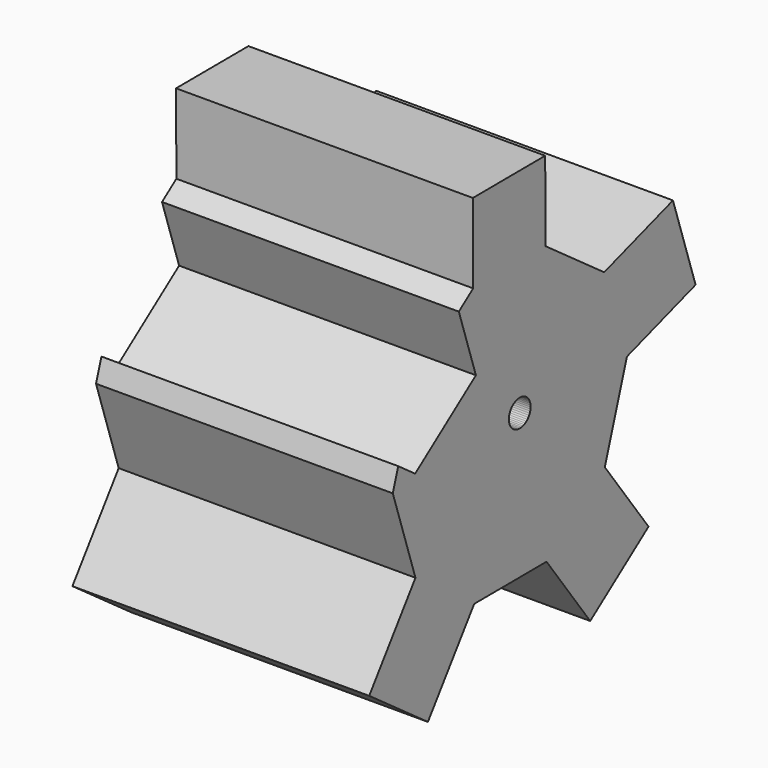
from build123d import *

# Parameters (mm, degrees)
F1_DEPTH = 59.967
F2_DEPTH = 16.11587
F3_DEPTH = 18.27724
F4_DEPTH = 18.65924
F5_DEPTH = 20.01095


with BuildPart() as f1:
    # F0 (on Right) → F1 (new body)
    with BuildSketch(Plane.YZ):
        Polygon((19.3016365517, 25.5114351168), (34.1311297964, 14.8414346621), (52.4001107586, 14.9257803925), (67.1304496505, 25.7322551057), (72.6956576812, 43.1331527599), (66.9700145375, 60.481921886), (52.1405212928, 71.1519223406), (33.8715403306, 71.0675766103), (30.248601096, 68.4097150693), (34.5660174948, 55.3278902953), (19.2159686951, 44.0667838525), (14.944761002, 47.1399696503), (13.575993408, 42.8602042428), align=None)
        Polygon((43.3843278169, 42.5439793365), (43.2058611327, 42.8390985452), (43.0657899565, 43.1542584575), (42.9663232941, 43.4844888132), (42.9090297944, 43.8245816823), (42.8948130101, 44.1691735971), (42.9238971483, 44.5128301373), (42.9958235348, 44.850131634), (43.1094578475, 45.175758641), (43.2630080055, 45.484575826), (43.454052431, 45.7717129574), (43.6795782392, 46.0326417111), (43.9360287536, 46.2632470849), (44.2193595962, 46.4598922942), (44.5251024704, 46.6194761267), (44.8484356285, 46.7394818499), (45.1842599134, 46.8180169019), (45.5272791756, 46.853842738), (45.8720837963, 46.8463943634), (46.2132360006, 46.7957892434), (46.5453556147, 46.7028254509), (46.8632049136, 46.5689690806), (47.1617712242, 46.3963311273), (47.4363459773, 46.1876341948), (47.6825989651, 45.9461695581), (47.8966466309, 45.6757452591), (48.075113315, 45.3806260503), (48.2151844913, 45.065466138), (48.3146511536, 44.7352357824), (48.3719446533, 44.3951429133), (48.3861614376, 44.0505509984), (48.3570772994, 43.7068944582), (48.2851509129, 43.3695929615), (48.1715166002, 43.0439659545), (48.0179664422, 42.7351487696), (47.8269220168, 42.4480116382), (47.6013962085, 42.1870828844), (47.3449456942, 41.9564775106), (47.0616148515, 41.7598323013), (46.7558719773, 41.6002484689), (46.4325388192, 41.4802427457), (46.0967145343, 41.4017076937), (45.7536952721, 41.3658818576), (45.4088906515, 41.3733302322), (45.0677384471, 41.4239353522), (44.7356188331, 41.5168991446), (44.4177695341, 41.6507555149), (44.1192032235, 41.8233934682), (43.8446284704, 42.0320904008), (43.5983754826, 42.2735550374), align=None, mode=Mode.SUBTRACT)
    extrude(amount=F1_DEPTH)

    # F2 (add): a face of the model
    f2_faces = [f1.faces().sort_by_distance(p)[0] for p in [
        (29.9835, 43.0060308117, 71.1097494755),
    ]]
    extrude(f2_faces, amount=F2_DEPTH)

    # F3 (add): a face of the model
    f3_faces = [f1.faces().sort_by_distance(p)[0] for p in [
        (29.9835, 69.8328361093, 51.8075373229),
    ]]
    extrude(f3_faces, amount=F3_DEPTH)

    # F4 (add): a face of the model
    f4_faces = [f1.faces().sort_by_distance(p)[0] for p in [
        (29.9835, 59.7652802045, 20.3290177491),
    ]]
    extrude(f4_faces, amount=F4_DEPTH)

    # F5 (add): a face of the model
    f5_faces = [f1.faces().sort_by_distance(p)[0] for p in [
        (29.9835, 26.7163831741, 20.1764348894),
    ]]
    extrude(f5_faces, amount=F5_DEPTH)


solid = f1.part
